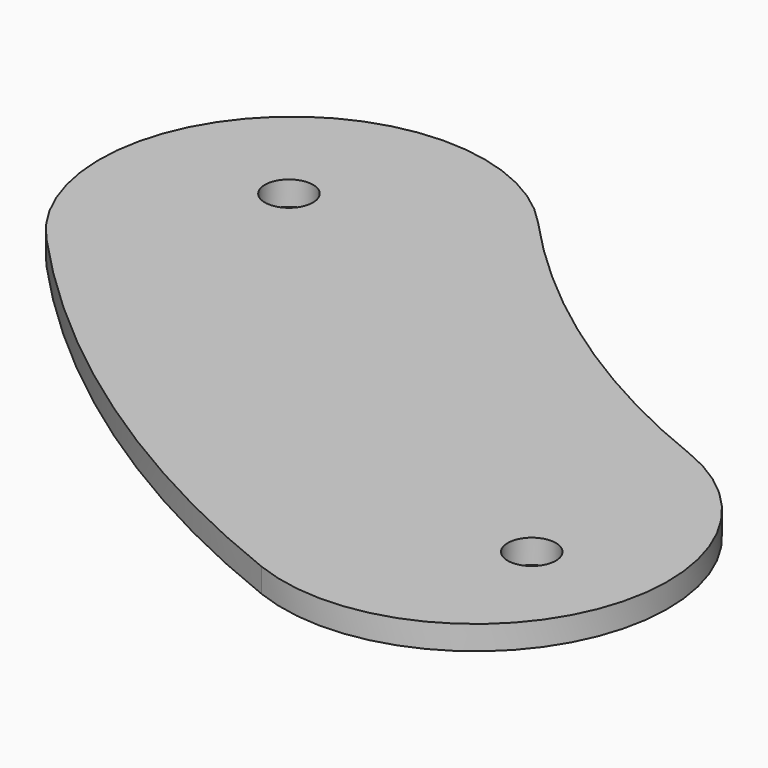
from build123d import *

# Parameters (mm, degrees)
F0_W     = 169.7224378586
F0_H     = 29.1480664164
F1_DEPTH = 5
F2_R     = 5
F3_DEPTH = 5.001
F6_R     = 5
F7_DEPTH = 5


# Not quite as in the source:
# - a feature of the source that left no trace in its solid (it failed there, or was rolled back) is left out


with BuildPart() as f1:
    # F0 (on Top) → F1 (new body)
    with BuildSketch(Plane.XY):
        with Locations((-209.8612189293, 14.5740332082)):
            Rectangle(F0_W, F0_H)
        Polygon((125, -249.6209740639), (125, -125), (-125, -125), (-125, 0), (-294.7224378586, 0), (-294.7224378586, -249.6209740639), align=None)
        Polygon((124.7859969735, -298.5799014568), (125, -249.6209740639), (-294.7224378586, -249.6209740639), (-294.7224378586, -298.5799014568), align=None)
    extrude(amount=F1_DEPTH)

    # F2 (on face) → F3 (cut, through all)
    with BuildSketch(Plane.XY.offset(5)):
        with Locations((-228.7230412454, -24.2026941362)):
            Circle(F2_R)
        with Locations((-219.7715429866, -67.8267564705)):
            Circle(F2_R)
        with Locations((-202.5809461153, -108.9080358424)):
            Circle(F2_R)
        with Locations((-177.7957154285, -145.9064206102)):
            Circle(F2_R)
        with Locations((-146.3450338267, -177.4348643144)):
            Circle(F2_R)
        with Locations((-109.4079678244, -202.3113851876)):
            Circle(F2_R)
        with Locations((-68.3692650785, -219.6033779172)):
            Circle(F2_R)
        with Locations((-24.7674410595, -228.6625764382)):
            Circle(F2_R)
        with Locations((19.7628989378, -229.1493570263)):
            Circle(F2_R)
        with Locations((63.5523401318, -221.0454705796)):
            Circle(F2_R)
    extrude(amount=-F3_DEPTH, mode=Mode.SUBTRACT)


with BuildPart() as f7:
    # F6 (on face) → F7 (new body)
    with BuildSketch(Plane.XY.offset(5)):
        with BuildLine():
            ThreePointArc((-44.6295934942, -213.8640500528), (-51.5484234193, -191.3776944906), (-69.9114028179, -176.6703024168))
            ThreePointArc((-69.9114028179, -176.6703024168), (-121.8233411216, -199.1458593545), (-99.3477842144, -251.0577976715))
            ThreePointArc((-99.3477842144, -251.0577976715), (-62.1432379515, -246.945220141), (-44.6295934942, -213.8640500528))
        make_face()
        with Locations((-109.4079678244, -202.3113851876)):
            Circle(F6_R, mode=Mode.SUBTRACT)
        with Locations((-68.3692650785, -219.6033779172)):
            Circle(F6_R, mode=Mode.SUBTRACT)
        with BuildLine():
            ThreePointArc((-139.8690317235, -128.5949220021), (-132.0468964749, -141.1390217828), (-129.3151434854, -155.6675373561))
            ThreePointArc((-129.3151434854, -155.6675373561), (-154.7866291142, -192.9357848352), (-198.7612569937, -182.7401508106))
            ThreePointArc((-198.7612569937, -182.7401508106), (-152.9185251389, -222.5217397679), (-99.3477842144, -251.0577976715))
            ThreePointArc((-99.3477842144, -251.0577976715), (-121.8233411216, -199.1458593545), (-69.9114028179, -176.6703024168))
            ThreePointArc((-69.9114028179, -176.6703024168), (-107.6093315173, -156.5893731081), (-139.8690317235, -128.5949220021))
        make_face()
        with BuildLine():
            ThreePointArc((-198.7612569937, -182.7401508106), (-154.7866291142, -192.9357848352), (-129.3151434854, -155.6675373561))
            ThreePointArc((-129.3151434854, -155.6675373561), (-132.0468964749, -141.1390217828), (-139.8690317235, -128.5949220021))
            ThreePointArc((-139.8690317235, -128.5949220021), (-196.3877578897, -126.221424721), (-198.7612569937, -182.7401508106))
        make_face()
        with Locations((-146.3450338267, -177.4348643144)):
            Circle(F6_R, mode=Mode.SUBTRACT)
        with Locations((-177.7957154285, -145.9064206102)):
            Circle(F6_R, mode=Mode.SUBTRACT)
        with Locations((-109.4079678244, -202.3113851876)):
            Circle(F6_R)
        with Locations((-146.3450338267, -177.4348643144)):
            Circle(F6_R)
    extrude(amount=F7_DEPTH)


solid = f7.part
